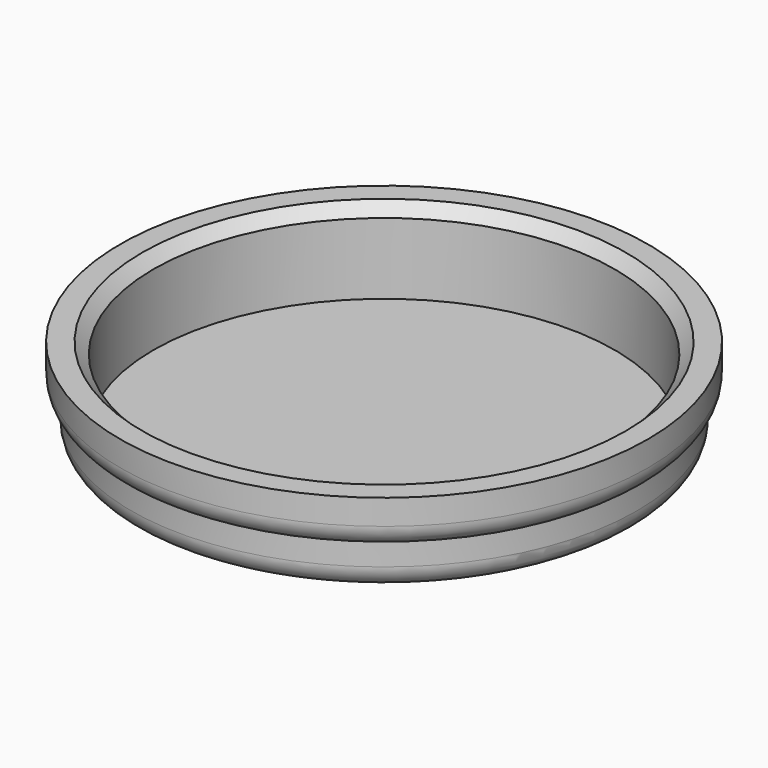
from build123d import *

# Parameters (mm, degrees)
F0_R     = 47.5
F0_R_2   = 41.5
F1_DEPTH = 16
F2_DEPTH = 1.2
F3_SIZE  = 2
F4_R     = 48.436615
F4_R_2   = 47.5
F4_R_3   = 45.5
F5_DEPTH = 8


# Not quite as in the source:
# - a fillet or chamfer that OpenCascade refuses, or shapes differently, is made with other operations: its cross-section is extruded or revolved along the edge and cut away or added


with BuildPart() as f1:
    # F0 (on Top) → F1 (new body)
    with BuildSketch(Plane.XY):
        Circle(F0_R)
        Circle(F0_R_2, mode=Mode.SUBTRACT)
    extrude(amount=F1_DEPTH)

    # F0 (on Top) → F2 (join)
    with BuildSketch(Plane.XY):
        Circle(F0_R_2)
    extrude(amount=F2_DEPTH)

    # F3
    f3_edges = [f1.edges().sort_by_distance(p)[0] for p in [
        (-41.5, 0, 16),
    ]]
    chamfer(f3_edges, length=F3_SIZE)

    # F4 (on face) → F5 (cut, symmetric)
    with BuildSketch(Plane(origin=(0, 0, 0), x_dir=(1, 0, 0), z_dir=(0, 0, -1))):
        Circle(F4_R)
        Circle(F4_R_2, mode=Mode.SUBTRACT)
        Circle(F4_R_2)
        Circle(F4_R_3, mode=Mode.SUBTRACT)
    extrude(amount=F5_DEPTH, both=True, mode=Mode.SUBTRACT)

    # F6: fillet of radius 4 on 2 edges, made by hand

    # F6_s1 → F6_t2 (revolve, cut)
    with BuildSketch(Plane.XZ):
        with BuildLine():
            ThreePointArc((47.5, 11.4641016151), (46.9641016151, 9.4641016151), (45.5, 8))
            Line((45.5, 8), (47.5, 8))
            Line((47.5, 8), (47.5, 11.4641016151))
        make_face()
    revolve(axis=Axis((0, 0, 8), (0, 0, -1)), mode=Mode.SUBTRACT)

    # F6_s3 → F6_t4 (revolve, cut)
    with BuildSketch(Plane.XZ):
        with BuildLine():
            ThreePointArc((45.5, 4), (44.3284271247, 1.1715728753), (41.5, 0))
            Line((41.5, 0), (45.5, 0))
            Line((45.5, 0), (45.5, 4))
        make_face()
    revolve(axis=Axis((0, 0, 0), (0, 0, 1)), mode=Mode.SUBTRACT)


solid = f1.part
